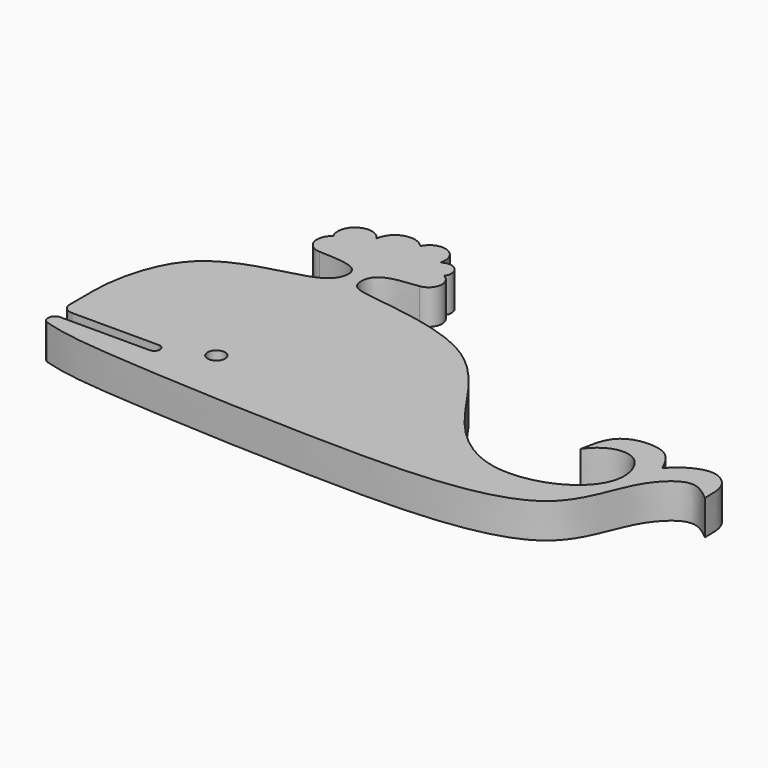
from build123d import *

# Parameters (mm, degrees)
F0_R     = 0.79375
F1_DEPTH = 3.175


with BuildPart() as f1:
    # F0 (on Top) → F1 (new body)
    with BuildSketch(Plane.XY):
        with BuildLine():
            Line((-12.1479392274, -1.3019143497), (-4.2125724058, -1.3019143497))
            ThreePointArc((-4.2125724058, -1.3019143497), (-3.6971087737, -1.8173779818), (-4.2125724058, -2.3328416139))
            Line((-4.2125724058, -2.3328416139), (-12.3618070082, -2.3328416139))
            ThreePointArc((-12.3618070082, -2.3328416139), (-12.9884320145, -2.8741308978), (-12.5439763069, -3.5727811046))
            add(Edge.make_bspline(
                [(-12.5439763069, -3.5727811046), (-10.4931714013, -4.1886749677), (-4.7138291604, -4.7848193904), (12.8140150399, -5.7225010361), (33.7629279781, -5.5893612026), (35.1803298379, 3.2155238376), (38.704793611, 6.4513086996), (40.2535807312, 5.1569357022), (40.9535728395, 4.5796856284)],
                knots=[0, 0, 0, 0, 0.1539240942, 0.4001297847, 0.6486499295, 0.8008356609, 0.9111762625, 1, 1, 1, 1], degree=3))
            add(Edge.make_bspline(
                [(40.9535728395, 4.5796856284), (40.965701297, 5.4104047878), (40.9891991521, 7.0198525291), (38.9013991928, 8.4470442608), (36.5460384231, 7.2291437108), (35.9495828805, 6.5502929537), (35.6991328299, 6.265245378)],
                knots=[0, 0, 0, 0, 0.2708933082, 0.5248327526, 0.8004785728, 1, 1, 1, 1], degree=3))
            add(Edge.make_bspline(
                [(29.298061505, 4.9477219582), (29.5057141134, 6.1436753777), (29.9264341111, 8.5667680789), (34.4643150607, 8.9013279289), (35.3069719217, 7.1024284451), (35.6991328299, 6.265245378)],
                knots=[0, 0, 0, 0, 0.3425496354, 0.6940316468, 1, 1, 1, 1], degree=3))
            add(Edge.make_bspline(
                [(4.6165669337, 17.4082815647), (3.2199198099, 17.2600813875), (0.919960215, 17.0320137683), (0.7655736955, 14.5125706311), (2.9776196983, 13.8268059586), (14.5338640425, 13.026433318), (19.5081363717, 2.7993005588), (25.5642344469, -1.8773343082), (32.1668367918, -0.6269388113), (35.0493534583, 3.0676669167), (33.2828979966, 7.258048808), (30.2664286615, 6.4002764567), (29.298061505, 4.9477219582)],
                knots=[0, 0, 0, 0, 0.0848731693, 0.1429757683, 0.2047674234, 0.352663907, 0.5035390936, 0.62458333, 0.7359914274, 0.8280273266, 0.9108507368, 1, 1, 1, 1], degree=3))
            ThreePointArc((4.6165669337, 17.4082815647), (5.6986880334, 18.4313854961), (4.9979779286, 19.7454376555))
            ThreePointArc((4.9979779286, 19.7454376555), (4.8579461757, 21.1161164274), (3.4805820532, 21.1512911574))
            ThreePointArc((3.4805820532, 21.1512911574), (2.6925940729, 23.0093893607), (0.8130051428, 22.2741346806))
            ThreePointArc((0.8130051428, 22.2741346806), (-1.1028000419, 22.7883978959), (-2.3620408028, 21.2557241321))
            ThreePointArc((-2.3620408028, 21.2557241321), (-4.4862537289, 21.7182494133), (-5.0077626444, 19.6077426869))
            ThreePointArc((-5.0077626444, 19.6077426869), (-5.5304899467, 18.0846492582), (-4.2496006936, 17.1087495983))
            add(Edge.make_bspline(
                [(-13.0761340261, 2.4947237689), (-13.0761340261, 4.3768916706), (-11.9038757056, 12.0029035771), (-2.6283669134, 13.2074512479), (-0.4747531489, 14.728784633), (-0.3660887841, 17.0050457573), (-2.880160515, 17.0732696657), (-4.2496006936, 17.1087495983)],
                knots=[0, 0, 0, 0, 0.2760675401, 0.5562594785, 0.7038936174, 0.8193056178, 1, 1, 1, 1], degree=3))
            Line((-13.0761340261, 2.4947237689), (-13.0761340261, -0.3737195511))
            ThreePointArc((-13.0761340261, -0.3737195511), (-12.8042720638, -1.0300523875), (-12.1479392274, -1.3019143497))
        make_face()
        Circle(F0_R, mode=Mode.SUBTRACT)
    extrude(amount=F1_DEPTH)


solid = f1.part
